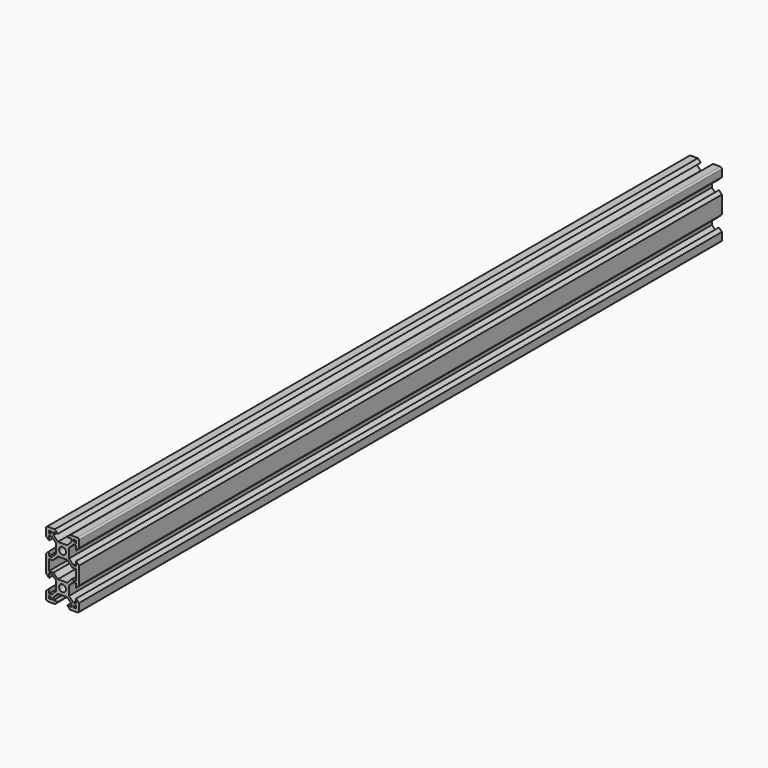
from build123d import *

# Parameters (mm, degrees)
F0_W             = 20
F0_H             = 20
F1_DEPTH         = 488
F2_R             = 2.1
F3_DEPTH         = 488.001
F4_R             = 1
F6_DEPTH         = 488.001
F6_COPIES3_COUNT = 2
F6_COPIES3_ANGLE = 90
F6_COPIES4_COUNT = 2
F6_COPIES4_ANGLE = 270
F6_COPIES6_COUNT = 2
F9_W             = 16.4
F9_H             = 6.8613203436
F10_DEPTH        = 488.001
F12_DEPTH        = 488


# Not quite as in the source:
# - a pattern or mirror of a feature is missing from the dataset's text; its kind, count and spacing are read off the source's solid


with BuildPart() as f1:
    # F0 (on Front) → F1 (new body)
    with BuildSketch(Plane.XZ):
        Rectangle(F0_W, F0_H)
    extrude(amount=F1_DEPTH)

    # F2 (on face) → F3 (cut, through all)
    with BuildSketch(Plane.XZ.offset(488)):
        Circle(F2_R)
    extrude(amount=-F3_DEPTH, mode=Mode.SUBTRACT)

    # F4
    f4_edges = [f1.edges().sort_by_distance(p)[0] for p in [
        (-10, -244, 10),
        (10, -244, 10),
    ]]
    fillet(f4_edges, radius=F4_R)

    # F5 (on face) → F6 (cut, through all)
    with BuildSketch(Plane.XZ.offset(488)):
        Polygon((0, 3.9006601718), (0, 10), (-2.84, 10), (-4.64, 10), (-2.84, 8.2), (-5.4993398282, 8.2), (-5.4993398282, 6.56), (-2.84, 3.9006601718), align=None)
        Polygon((-6.5693398282, 8.2), (-8.2, 8.2), (-7.0953059148, 7.0953059148), (-6.5693398282, 7.6212720014), align=None)
    f6 = extrude(amount=-F6_DEPTH, mode=Mode.SUBTRACT)

    # F6_copies: F6 across plane
    add(f6.mirror(Plane(origin=(0, 0, 0), x_dir=(-0.7071067812, 0, -0.7071067812), z_dir=(0.7071067812, 0, -0.7071067812))), mode=Mode.SUBTRACT)

    # F6_copies1: F6 across plane
    add(f6.mirror(Plane(origin=(0, 0, 0), x_dir=(0.7071067812, 0, -0.7071067812), z_dir=(-0.7071067812, 0, -0.7071067812))), mode=Mode.SUBTRACT)

    # F6_copies2: F6 across plane
    add(f6.mirror(Plane(origin=(0, 0, 0), x_dir=(0, 0, 1), z_dir=(1, 0, 0))), mode=Mode.SUBTRACT)

    # F6_copies3: F6 ×2 about axis
    f6_copies3_axis = Axis((0, 0, 0), (0, 1, 0))
    for i in range(1, F6_COPIES3_COUNT):
        add(f6.rotate(f6_copies3_axis, i * F6_COPIES3_ANGLE / (F6_COPIES3_COUNT - 1)), mode=Mode.SUBTRACT)

    # F6_copies4: F6 ×2 about axis
    f6_copies4_axis = Axis((0, 0, 0), (0, 1, 0))
    for i in range(1, F6_COPIES4_COUNT):
        add(f6.rotate(f6_copies4_axis, i * F6_COPIES4_ANGLE / (F6_COPIES4_COUNT - 1)), mode=Mode.SUBTRACT)

    # F6_copies5: F6 across plane
    add(f6.mirror(Plane(origin=(0, 0, 0), x_dir=(-1, 0, 0), z_dir=(0, 0, -1))), mode=Mode.SUBTRACT)

    # F6_copies6: F6 ×2 about axis
    f6_copies6_axis = Axis((0, 0, 0), (0, 1, 0))
    for i in range(1, F6_COPIES6_COUNT):
        add(f6.rotate(f6_copies6_axis, i * 360 / F6_COPIES6_COUNT), mode=Mode.SUBTRACT)

    # F8: F1 across face


with BuildPart() as f1_1:
    add(f1.part)
    add(f1.part.mirror(Plane(origin=(-7.32, -244, -10), x_dir=(1, 0, 0), z_dir=(0, 0, -1))))

    # F9 (on face) → F10 (cut, through all)
    with BuildSketch(Plane.XZ.offset(488)):
        with Locations((0, -10)):
            Rectangle(F9_W, F9_H)
    extrude(amount=-F10_DEPTH, mode=Mode.SUBTRACT)

    # F11 (on face) → F12 (join, through all)
    with BuildSketch(Plane.XZ.offset(488)):
        with BuildLine():
            ThreePointArc((-9, -10), (-9.7071067812, -9.7071067812), (-10, -9))
            Line((-10, -9), (-10, -11))
            ThreePointArc((-10, -11), (-9.7071067812, -10.2928932188), (-9, -10))
        make_face()
        with BuildLine():
            ThreePointArc((10, -9), (9.7071067812, -9.7071067812), (9, -10))
            ThreePointArc((9, -10), (9.7071067812, -10.2928932188), (10, -11))
            Line((10, -11), (10, -9))
        make_face()
        Polygon((5.9386796564, -6.9993398282), (8.2, -6.9993398282), (8.2, -6.5693398282), (5.5086796564, -6.5693398282), align=None)
        Polygon((-8.2, -6.5693398282), (-8.2, -6.9993398282), (-5.9386796564, -6.9993398282), (-5.5086796564, -6.5693398282), align=None)
    extrude(amount=-F12_DEPTH)


solid = f1_1.part
